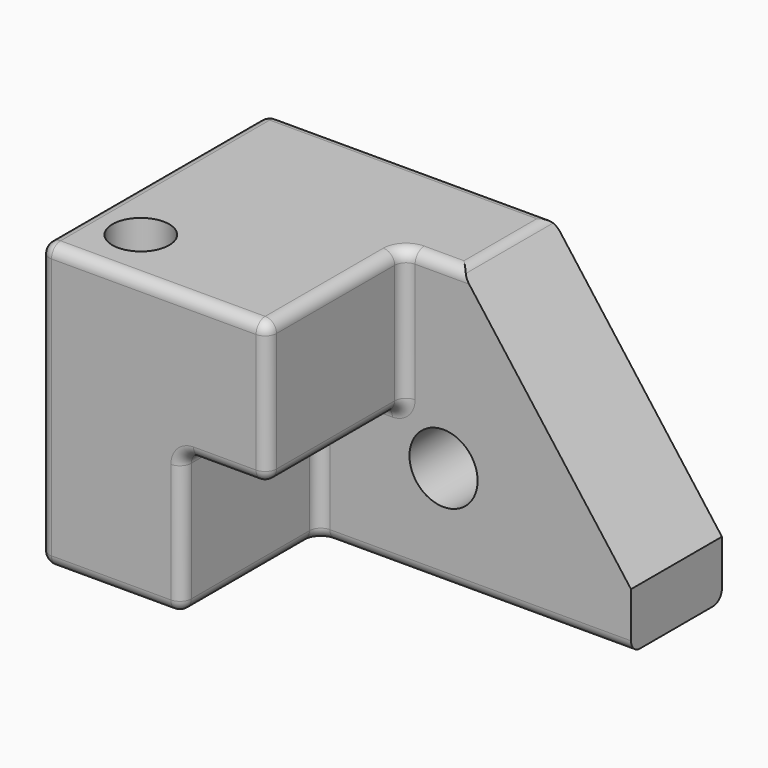
from build123d import *

# Parameters (mm, degrees)
F1_DEPTH = 127
F3_DEPTH = 76.2
F4_SIZE2 = 101.6
F4_SIZE  = 76.2
F5_R     = 5.08
F6_R     = 15.24
F7_DEPTH = 50.8
F8_R     = 12.7
F9_DEPTH = 127


with BuildPart() as f1:
    # F0 (on Front) → F1 (new body)
    with BuildSketch(Plane.XZ):
        Polygon((-38.1, -63.5), (101.6, -63.5), (101.6, 63.5), (0, 63.5), (0, 0), (-38.1, 0), align=None)
        Polygon((-101.6, -63.5), (-38.1, -63.5), (-38.1, 0), (0, 0), (0, 63.5), (-101.6, 63.5), align=None)
    extrude(amount=F1_DEPTH)

    # F2 (on face) → F3 (cut)
    with BuildSketch(Plane.XZ.offset(127)):
        Polygon((-38.1, 0), (-38.1, -63.5), (101.6, -63.5), (101.6, 63.5), (0, 63.5), (0, 0), align=None)
    extrude(amount=-F3_DEPTH, mode=Mode.SUBTRACT)

    # F4
    f4_edges = [f1.edges().sort_by_distance(p)[0] for p in [
        (101.6, -25.4, 63.5),
    ]]
    f4_side = f1.faces().sort_by_distance((-21.771429, -52.614286, 63.5))[0]
    chamfer(f4_edges, length=F4_SIZE, length2=F4_SIZE2, reference=f4_side)

    # F5
    f5_edges = [f1.edges().sort_by_distance(p)[0] for p in [
        (12.7, -50.8, 63.5),
        (25.4, -25.4, 63.5),
        (0, -88.9, 63.5),
        (-50.8, -127, 63.5),
        (0, -127, 31.75),
        (0, -88.9, 0),
        (-19.05, -127, 0),
        (-38.1, -127, -31.75),
        (-38.1, -88.9, -63.5),
        (-69.85, -127, -63.5),
        (-101.6, -127, 0),
        (-101.6, -63.5, 63.5),
        (-38.1, 0, 63.5),
        (-38.1, -50.8, -31.75),
        (-38.1, -88.9, 0),
        (-19.05, -50.8, 0),
        (-101.6, 0, 0),
        (-101.6, -63.5, -63.5),
        (0, 0, -63.5),
        (31.75, -50.8, -63.5),
        (0, -50.8, 31.75),
    ]]
    fillet(f5_edges, radius=F5_R)

    # F6 (on face) → F7 (cut, through all)
    with BuildSketch(Plane.XZ.offset(50.8)):
        with Locations((17.78, -17.78)):
            Circle(F6_R)
    extrude(amount=-F7_DEPTH, mode=Mode.SUBTRACT)

    # F8 (on face) → F9 (cut, through all)
    with BuildSketch(Plane.XY.offset(63.5)):
        with Locations((-77.5449126959, -100.8186563849)):
            Circle(F8_R)
    extrude(amount=-F9_DEPTH, mode=Mode.SUBTRACT)


solid = f1.part
